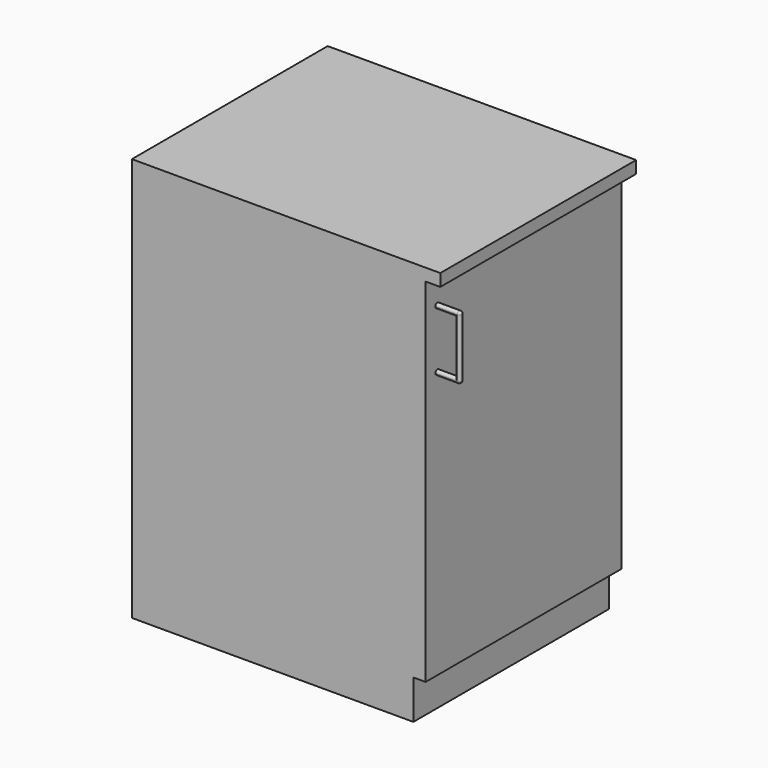
from build123d import *

# Parameters (mm, degrees)
F0_W        = 600
F0_H        = 500
F1_DEPTH    = 800
F2_W        = 500
F2_H        = 80
F3_DEPTH    = 25
F5_DEPTH    = 50
F6_T1_DEPTH = 120
F6_T4_ANGLE = 180
F6_T6_ANGLE = 180
F7_W        = 40
F7_H        = 110
F8_DEPTH    = 25
F9_R        = 4.99999
F10_W       = 630
F10_H       = 500
F11_DEPTH   = 25


# Not quite as in the source:
# - a fillet or chamfer that OpenCascade refuses, or shapes differently, is made with other operations: its cross-section is extruded or revolved along the edge and cut away or added
# - a fillet or chamfer is up to 0.001 mm smaller than in the source, because OpenCascade refuses the exact size


with BuildPart() as f1:
    # F0 (on Top) → F1 (new body)
    with BuildSketch(Plane.XY):
        Rectangle(F0_W, F0_H)
    extrude(amount=F1_DEPTH)

    # F2 (on face) → F3 (cut)
    with BuildSketch(Plane.YZ.offset(300)):
        with Locations((0, 40)):
            Rectangle(F2_W, F2_H)
    extrude(amount=-F3_DEPTH, mode=Mode.SUBTRACT)

    # F4 (on face) → F5 (join)
    with BuildSketch(Plane.YZ.offset(300)):
        with BuildLine():
            ThreePointArc((-220, 750), (-223.5355339059, 748.5355339059), (-225, 745))
            Line((-225, 745), (-225, 625))
            ThreePointArc((-225, 625), (-223.5355339059, 621.4644660941), (-220, 620))
            ThreePointArc((-220, 620), (-216.4644660941, 621.4644660941), (-215, 625))
            Line((-215, 625), (-215, 745))
            ThreePointArc((-215, 745), (-216.4644660941, 748.5355339059), (-220, 750))
        make_face()
    extrude(amount=F5_DEPTH)

    # F6: fillet of radius 5 on 4 edges, made by hand

    # F6_s2 → F6_t1 (cut)
    with BuildSketch(Plane.XY.offset(625)):
        with BuildLine():
            ThreePointArc((345, -225), (348.5355339059, -223.5355339059), (350, -220))
            Line((350, -220), (350.1, -220))
            Line((350.1, -220), (350.1, -225.1))
            Line((350.1, -225.1), (345, -225.1))
            Line((345, -225.1), (345, -225))
        make_face()
        with BuildLine():
            ThreePointArc((345, -215), (348.5355339059, -216.4644660941), (350, -220))
            Line((350, -220), (350.1, -220))
            Line((350.1, -220), (350.1, -214.9))
            Line((350.1, -214.9), (345, -214.9))
            Line((345, -214.9), (345, -215))
        make_face()
    extrude(amount=F6_T1_DEPTH, mode=Mode.SUBTRACT)

    # F6_s3 → F6_t4 (revolve, cut)
    with BuildSketch(Plane.XY.offset(745)):
        with BuildLine():
            ThreePointArc((345, -225), (348.5355339059, -223.5355339059), (350, -220))
            Line((350, -220), (350.1, -220))
            Line((350.1, -220), (350.1, -225.1))
            Line((350.1, -225.1), (345, -225.1))
            Line((345, -225.1), (345, -225))
        make_face()
    revolve(axis=Axis((350, -220, 745), (-1, 0, 0)), revolution_arc=F6_T4_ANGLE, mode=Mode.SUBTRACT)

    # F6_s5 → F6_t6 (revolve, cut)
    with BuildSketch(Plane.XY.offset(625)):
        with BuildLine():
            ThreePointArc((345, -215), (348.5355339059, -216.4644660941), (350, -220))
            Line((350, -220), (350.1, -220))
            Line((350.1, -220), (350.1, -214.9))
            Line((350.1, -214.9), (345, -214.9))
            Line((345, -214.9), (345, -215))
        make_face()
    revolve(axis=Axis((350, -220, 625), (-1, 0, 0)), revolution_arc=F6_T6_ANGLE, mode=Mode.SUBTRACT)

    # F7 (on face) → F8 (cut)
    with BuildSketch(Plane(origin=(0, -215, 0), x_dir=(-1, 0, 0), z_dir=(0, 1, 0))):
        with Locations((-320, 685)):
            Rectangle(F7_W, F7_H)
    extrude(amount=-F8_DEPTH, mode=Mode.SUBTRACT)

    # F9 (radius 5 in the source; OpenCascade refuses exactly that, so slightly less here)
    f9_edges = [f1.edges().sort_by_distance(p)[0] for p in [
        (320, -215, 740),
        (340, -215, 685),
        (320, -215, 630),
        (320, -225, 740),
        (340, -225, 685),
        (320, -225, 630),
    ]]
    fillet(f9_edges, radius=F9_R)

    # F10 (on face) → F11 (join)
    with BuildSketch(Plane.XY.offset(800)):
        with Locations((15, 0)):
            Rectangle(F10_W, F10_H)
    extrude(amount=F11_DEPTH)


solid = f1.part
